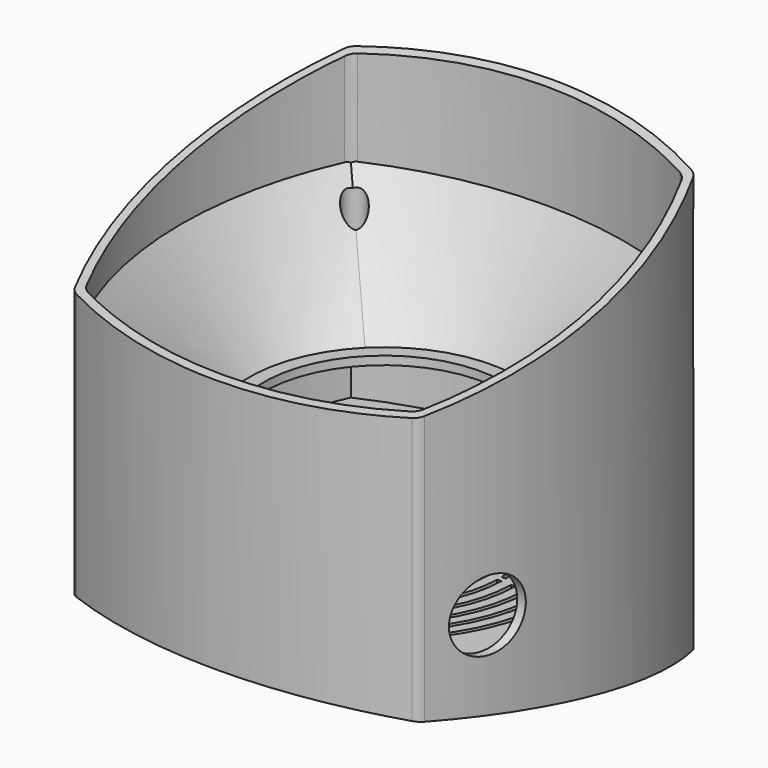
from build123d import *

# Parameters (mm, degrees)
F1_DEPTH        = 80
F2_R            = 1379.3418086479
F3_DEPTH        = 390
F0_R            = 47.8625
F7_DEPTH        = 40
F8_R            = 47.8625
F10_R           = 42.8625
F11_DEPTH       = 3
F14_DEPTH       = 31
F16_DEPTH       = 25
F17_R           = 5
F20_D           = 4
F20_START       = 24.8328661
F20_CBORE_D     = 8
F20_CBORE_DEPTH = 5
F21_R           = 2
F22_DEPTH       = 3
F23_R           = 12.5
F24_DEPTH       = 249


# Not quite as in the source:
# - a feature names something its author has since deleted; it is built from what else it names


with BuildPart() as f1:
    # F0 (on Top) → F1 (new body, symmetric)
    with BuildSketch(Plane.XY):
        with BuildLine():
            ThreePointArc((61.2553872941, -61.2553872941), (75.039376183, 0), (61.2553872941, 61.2553872941))
            ThreePointArc((61.2553872941, 61.2553872941), (0, 75.039376183), (-61.2553872941, 61.2553872941))
            ThreePointArc((-61.2553872941, 61.2553872941), (-75.039376183, 0), (-61.2553872941, -61.2553872941))
            ThreePointArc((-61.2553872941, -61.2553872941), (0, -75.039376183), (61.2553872941, -61.2553872941))
        make_face()
        with BuildLine():
            ThreePointArc((-59, 59), (0, 72.039376183), (59, 59))
            ThreePointArc((59, 59), (72.039376183, 0), (59, -59))
            ThreePointArc((59, -59), (0, -72.039376183), (-59, -59))
            ThreePointArc((-59, -59), (-72.039376183, 0), (-59, 59))
        make_face(mode=Mode.SUBTRACT)
    extrude(amount=F1_DEPTH, both=True)

    # F2 (on Right) → F3 (cut, symmetric)
    with BuildSketch(Plane.YZ):
        with Locations((-294.0411567688, 1407.0612192154)):
            Circle(F2_R)
        with Locations((-294.0411567688, -1407.0612192154)):
            Circle(F2_R)
    extrude(amount=F3_DEPTH, both=True, mode=Mode.SUBTRACT)

    # F6 (on Top) + F0 (on Top) → F7 (join, symmetric)
    with BuildSketch(Plane.XY):
        with BuildLine():
            ThreePointArc((61.2553872941, -61.2553872941), (75.039376183, 0), (61.2553872941, 61.2553872941))
            ThreePointArc((61.2553872941, 61.2553872941), (0, 75.039376183), (-61.2553872941, 61.2553872941))
            ThreePointArc((-61.2553872941, 61.2553872941), (-75.039376183, 0), (-61.2553872941, -61.2553872941))
            ThreePointArc((-61.2553872941, -61.2553872941), (0, -75.039376183), (61.2553872941, -61.2553872941))
        make_face()
        with BuildLine():
            ThreePointArc((-59, 59), (0, 72.039376183), (59, 59))
            ThreePointArc((59, 59), (72.039376183, 0), (59, -59))
            ThreePointArc((59, -59), (0, -72.039376183), (-59, -59))
            ThreePointArc((-59, -59), (-72.039376183, 0), (-59, 59))
        make_face(mode=Mode.SUBTRACT)
        with BuildLine():
            ThreePointArc((59, -59), (72.039376183, 0), (59, 59))
            ThreePointArc((59, 59), (0, 72.039376183), (-59, 59))
            ThreePointArc((-59, 59), (-72.039376183, 0), (-59, -59))
            ThreePointArc((-59, -59), (0, -72.039376183), (59, -59))
        make_face()
    with BuildSketch(Plane.XY):
        with BuildLine():
            ThreePointArc((59, -59), (72.039376183, 0), (59, 59))
            ThreePointArc((59, 59), (0, 72.039376183), (-59, 59))
            ThreePointArc((-59, 59), (-72.039376183, 0), (-59, -59))
            ThreePointArc((-59, -59), (0, -72.039376183), (59, -59))
        make_face()
        Circle(F0_R, mode=Mode.SUBTRACT)
    extrude(amount=F7_DEPTH, both=True)

    # F5 (on offset) → F9 section 0
    with BuildSketch(Plane.XY.offset(40)):
        with BuildLine():
            ThreePointArc((59, -59), (72.039376183, 0), (59, 59))
            ThreePointArc((59, 59), (0, 72.039376183), (-59, 59))
            ThreePointArc((-59, 59), (-72.039376183, 0), (-59, -59))
            ThreePointArc((-59, -59), (0, -72.039376183), (59, -59))
        make_face()
    # F8 (on Top) → F9 section 1
    with BuildSketch(Plane.XY):
        Circle(F8_R)
    loft(mode=Mode.SUBTRACT)

    # F10 (on face) → F11 (cut)
    with BuildSketch(Plane.XY):
        Circle(F10_R)
    extrude(amount=-F11_DEPTH, mode=Mode.SUBTRACT)

    # F13 (on offset) → F14 (cut)
    with BuildSketch(Plane.XY.offset(-3)):
        with BuildLine():
            ThreePointArc((59, -59), (72.039376183, 0), (59, 59))
            ThreePointArc((59, 59), (0, 72.039376183), (-59, 59))
            ThreePointArc((-59, 59), (-72.039376183, 0), (-59, -59))
            ThreePointArc((-59, -59), (0, -72.039376183), (59, -59))
        make_face()
    extrude(amount=-F14_DEPTH, mode=Mode.SUBTRACT)

    # F15 (on face) → F16 (cut)
    with BuildSketch(Plane(origin=(0, 0, -40), x_dir=(1, 0, 0), z_dir=(0, 0, -1))):
        with BuildLine():
            Line((-1, 60.9918027279), (-1, 62.4919994879))
            ThreePointArc((-1, 62.4919994879), (-44.1941738242, 44.1941738242), (-62.4919994879, 1))
            Line((-62.4919994879, 1), (-60.9918027279, 1))
            ThreePointArc((-60.9918027279, 1), (-43.1335136524, 43.1335136524), (-1, 60.9918027279))
        make_face()
        with BuildLine():
            Line((-1, 55.9910707167), (-1, 57.4913036902))
            ThreePointArc((-1, 57.4913036902), (-40.6586399182, 40.6586399182), (-57.4913036902, 1))
            Line((-57.4913036902, 1), (-55.9910707167, 1))
            ThreePointArc((-55.9910707167, 1), (-39.5979797464, 39.5979797464), (-1, 55.9910707167))
        make_face()
        with BuildLine():
            Line((-1, 50.9901951359), (-1, 52.4904753265))
            ThreePointArc((-1, 52.4904753265), (-37.1231060123, 37.1231060123), (-52.4904753265, 1))
            Line((-52.4904753265, 1), (-50.9901951359, 1))
            ThreePointArc((-50.9901951359, 1), (-36.0624458405, 36.0624458405), (-1, 50.9901951359))
        make_face()
        with BuildLine():
            Line((-1, 45.9891291503), (-1, 47.4894725176))
            ThreePointArc((-1, 47.4894725176), (-33.5875721064, 33.5875721064), (-47.4894725176, 1))
            Line((-47.4894725176, 1), (-45.9891291503, 1))
            ThreePointArc((-45.9891291503, 1), (-32.5269119346, 32.5269119346), (-1, 45.9891291503))
        make_face()
        with BuildLine():
            Line((-1, 40.9878030638), (-1, 42.4882336653))
            ThreePointArc((-1, 42.4882336653), (-30.0520382004, 30.0520382004), (-42.4882336653, 1))
            Line((-42.4882336653, 1), (-40.9878030638, 1))
            ThreePointArc((-40.9878030638, 1), (-28.9913780286, 28.9913780286), (-1, 40.9878030638))
        make_face()
        with BuildLine():
            Line((-1, 35.9861084309), (-1, 37.4866642955))
            ThreePointArc((-1, 37.4866642955), (-26.5165042945, 26.5165042945), (-37.4866642955, 1))
            Line((-37.4866642955, 1), (-35.9861084309, 1))
            ThreePointArc((-35.9861084309, 1), (-25.4558441227, 25.4558441227), (-1, 35.9861084309))
        make_face()
        with BuildLine():
            Line((35.9861084309, 1), (37.4866642955, 1))
            ThreePointArc((37.4866642955, 1), (26.5165042945, 26.5165042945), (1, 37.4866642955))
            Line((1, 37.4866642955), (1, 35.9861084309))
            ThreePointArc((1, 35.9861084309), (25.4558441227, 25.4558441227), (35.9861084309, 1))
        make_face()
        with BuildLine():
            Line((40.9878030638, 1), (42.4882336653, 1))
            ThreePointArc((42.4882336653, 1), (30.0520382004, 30.0520382004), (1, 42.4882336653))
            Line((1, 42.4882336653), (1, 40.9878030638))
            ThreePointArc((1, 40.9878030638), (28.9913780286, 28.9913780286), (40.9878030638, 1))
        make_face()
        with BuildLine():
            Line((45.9891291503, 1), (47.4894725176, 1))
            ThreePointArc((47.4894725176, 1), (33.5875721064, 33.5875721064), (1, 47.4894725176))
            Line((1, 47.4894725176), (1, 45.9891291503))
            ThreePointArc((1, 45.9891291503), (32.5269119346, 32.5269119346), (45.9891291503, 1))
        make_face()
        with BuildLine():
            Line((50.9901951359, 1), (52.4904753265, 1))
            ThreePointArc((52.4904753265, 1), (37.1231060123, 37.1231060123), (1, 52.4904753265))
            Line((1, 52.4904753265), (1, 50.9901951359))
            ThreePointArc((1, 50.9901951359), (36.0624458405, 36.0624458405), (50.9901951359, 1))
        make_face()
        with BuildLine():
            Line((55.9910707167, 1), (57.4913036902, 1))
            ThreePointArc((57.4913036902, 1), (40.6586399182, 40.6586399182), (1, 57.4913036902))
            Line((1, 57.4913036902), (1, 55.9910707167))
            ThreePointArc((1, 55.9910707167), (39.5979797464, 39.5979797464), (55.9910707167, 1))
        make_face()
        with BuildLine():
            Line((60.9918027279, 1), (62.4919994879, 1))
            ThreePointArc((62.4919994879, 1), (44.1941738242, 44.1941738242), (1, 62.4919994879))
            Line((1, 62.4919994879), (1, 60.9918027279))
            ThreePointArc((1, 60.9918027279), (43.1335136524, 43.1335136524), (60.9918027279, 1))
        make_face()
        with BuildLine():
            ThreePointArc((1, -37.4866642955), (26.5165042945, -26.5165042945), (37.4866642955, -1))
            Line((37.4866642955, -1), (35.9861084309, -1))
            ThreePointArc((35.9861084309, -1), (25.4558441227, -25.4558441227), (1, -35.9861084309))
            Line((1, -35.9861084309), (1, -37.4866642955))
        make_face()
        with BuildLine():
            ThreePointArc((-37.4866642955, -1), (-26.5165042945, -26.5165042945), (-1, -37.4866642955))
            Line((-1, -37.4866642955), (-1, -35.9861084309))
            ThreePointArc((-1, -35.9861084309), (-25.4558441227, -25.4558441227), (-35.9861084309, -1))
            Line((-35.9861084309, -1), (-37.4866642955, -1))
        make_face()
        with BuildLine():
            ThreePointArc((-42.4882336653, -1), (-30.0520382004, -30.0520382004), (-1, -42.4882336653))
            Line((-1, -42.4882336653), (-1, -40.9878030638))
            ThreePointArc((-1, -40.9878030638), (-28.9913780286, -28.9913780286), (-40.9878030638, -1))
            Line((-40.9878030638, -1), (-42.4882336653, -1))
        make_face()
        with BuildLine():
            ThreePointArc((1, -42.4882336653), (30.0520382004, -30.0520382004), (42.4882336653, -1))
            Line((42.4882336653, -1), (40.9878030638, -1))
            ThreePointArc((40.9878030638, -1), (28.9913780286, -28.9913780286), (1, -40.9878030638))
            Line((1, -40.9878030638), (1, -42.4882336653))
        make_face()
        with BuildLine():
            ThreePointArc((1, -47.4894725176), (33.5875721064, -33.5875721064), (47.4894725176, -1))
            Line((47.4894725176, -1), (45.9891291503, -1))
            ThreePointArc((45.9891291503, -1), (32.5269119346, -32.5269119346), (1, -45.9891291503))
            Line((1, -45.9891291503), (1, -47.4894725176))
        make_face()
        with BuildLine():
            ThreePointArc((-47.4894725176, -1), (-33.5875721064, -33.5875721064), (-1, -47.4894725176))
            Line((-1, -47.4894725176), (-1, -45.9891291503))
            ThreePointArc((-1, -45.9891291503), (-32.5269119346, -32.5269119346), (-45.9891291503, -1))
            Line((-45.9891291503, -1), (-47.4894725176, -1))
        make_face()
        with BuildLine():
            ThreePointArc((-52.4904753265, -1), (-37.1231060123, -37.1231060123), (-1, -52.4904753265))
            Line((-1, -52.4904753265), (-1, -50.9901951359))
            ThreePointArc((-1, -50.9901951359), (-36.0624458405, -36.0624458405), (-50.9901951359, -1))
            Line((-50.9901951359, -1), (-52.4904753265, -1))
        make_face()
        with BuildLine():
            ThreePointArc((1, -52.4904753265), (37.1231060123, -37.1231060123), (52.4904753265, -1))
            Line((52.4904753265, -1), (50.9901951359, -1))
            ThreePointArc((50.9901951359, -1), (36.0624458405, -36.0624458405), (1, -50.9901951359))
            Line((1, -50.9901951359), (1, -52.4904753265))
        make_face()
        with BuildLine():
            ThreePointArc((1, -57.4913036902), (40.6586399182, -40.6586399182), (57.4913036902, -1))
            Line((57.4913036902, -1), (55.9910707167, -1))
            ThreePointArc((55.9910707167, -1), (39.5979797464, -39.5979797464), (1, -55.9910707167))
            Line((1, -55.9910707167), (1, -57.4913036902))
        make_face()
        with BuildLine():
            ThreePointArc((-57.4913036902, -1), (-40.6586399182, -40.6586399182), (-1, -57.4913036902))
            Line((-1, -57.4913036902), (-1, -55.9910707167))
            ThreePointArc((-1, -55.9910707167), (-39.5979797464, -39.5979797464), (-55.9910707167, -1))
            Line((-55.9910707167, -1), (-57.4913036902, -1))
        make_face()
        with BuildLine():
            ThreePointArc((-62.4919994879, -1), (-44.1941738242, -44.1941738242), (-1, -62.4919994879))
            Line((-1, -62.4919994879), (-1, -60.9918027279))
            ThreePointArc((-1, -60.9918027279), (-43.1335136524, -43.1335136524), (-60.9918027279, -1))
            Line((-60.9918027279, -1), (-62.4919994879, -1))
        make_face()
        with BuildLine():
            ThreePointArc((1, -62.4919994879), (44.1941738242, -44.1941738242), (62.4919994879, -1))
            Line((62.4919994879, -1), (60.9918027279, -1))
            ThreePointArc((60.9918027279, -1), (43.1335136524, -43.1335136524), (1, -60.9918027279))
            Line((1, -60.9918027279), (1, -62.4919994879))
        make_face()
    extrude(amount=-F16_DEPTH, mode=Mode.SUBTRACT)

    # F17
    f17_edges = [f1.edges().sort_by_distance(p)[0] for p in [
        (-61.255387, 61.255387, 0),
        (-61.255387, -61.255387, 0),
        (61.255387, 61.255387, 0),
        (61.255387, -61.255387, 0),
        (-59, 59, 56.832446),
        (59, 59, 56.832446),
        (-59, -59, 43.946273),
        (59, -59, 43.946273),
        (59, -59, -43.946273),
        (-59, -59, -43.946273),
        (-59, 59, -56.832446),
        (59, 59, -56.832446),
    ]]
    fillet(f17_edges, radius=F17_R)

    # F20 (through all)
    # its depths count from where the whole tool has entered the part; down to there all is cleared
    with Locations(Plane.XY.offset(50).offset(-F20_START)):
        with Locations((-52.5, 52.5), (52.5, 52.5), (52.5, -52.5), (-52.5, -52.5)):
            CounterBoreHole(F20_D / 2, F20_CBORE_D / 2, F20_CBORE_DEPTH)

    # F21 (on face) → F22 (cut)
    with BuildSketch(Plane(origin=(0, 0, -40), x_dir=(1, 0, 0), z_dir=(0, 0, -1))):
        Polygon((-50.7679491924, 55.5), (-54.2320508076, 55.5), (-55.9641016151, 52.5), (-54.2320508076, 49.5), (-50.7679491924, 49.5), (-49.0358983849, 52.5), align=None)
        with Locations((-52.5, 52.5)):
            Circle(F21_R, mode=Mode.SUBTRACT)
        Polygon((54.2320508076, 55.5), (50.7679491924, 55.5), (49.0358983849, 52.5), (50.7679491924, 49.5), (54.2320508076, 49.5), (55.9641016151, 52.5), align=None)
        with Locations((52.5, 52.5)):
            Circle(F21_R, mode=Mode.SUBTRACT)
        Polygon((54.2320508076, -49.5), (50.7679491924, -49.5), (49.0358983849, -52.5), (50.7679491924, -55.5), (54.2320508076, -55.5), (55.9641016151, -52.5), align=None)
        with Locations((52.5, -52.5)):
            Circle(F21_R, mode=Mode.SUBTRACT)
        Polygon((-50.7679491924, -49.5), (-54.2320508076, -49.5), (-55.9641016151, -52.5), (-54.2320508076, -55.5), (-50.7679491924, -55.5), (-49.0358983849, -52.5), align=None)
        with Locations((-52.5, -52.5)):
            Circle(F21_R, mode=Mode.SUBTRACT)
    extrude(amount=-F22_DEPTH, mode=Mode.SUBTRACT)

    # F23 (on Right) → F24 (cut)
    with BuildSketch(Plane.YZ):
        with Locations((-40, -20)):
            Circle(F23_R)
    extrude(amount=F24_DEPTH, mode=Mode.SUBTRACT)


solid = f1.part
